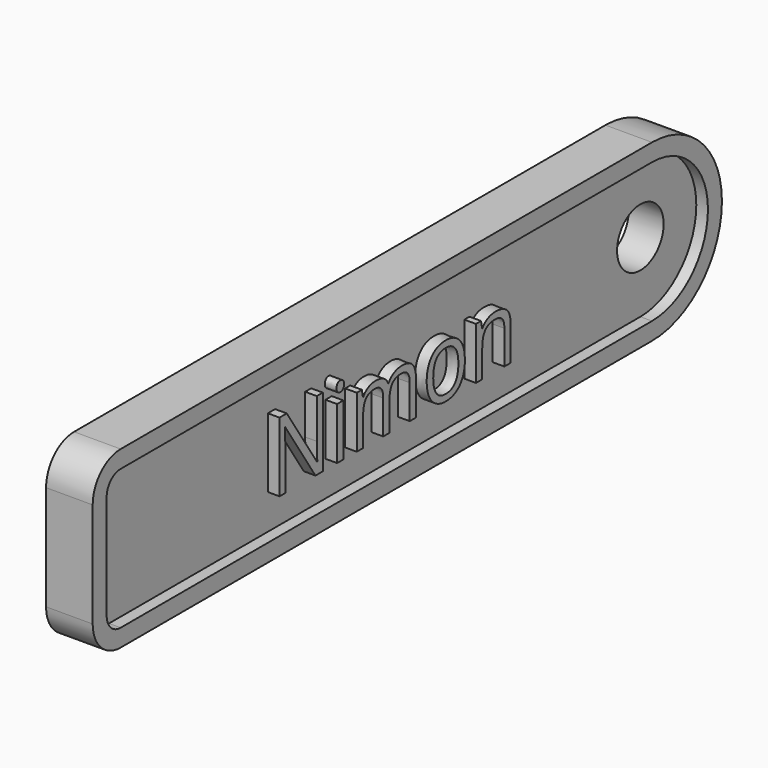
from build123d import *

# Parameters (mm, degrees)
F0_R         = 63.5
F1_DEPTH     = 76.2
F2_TEXT_SIZE = 211.6666666667
F3_DEPTH     = 25.4
F5_DEPTH     = 25.4


# Not quite as in the source:
# - Text() gives the source's letters only with a copy of the font that has no kerning and outlines rounded to 1/6400 em; it was checked with that copy


with BuildPart() as f1:
    # F0 (on Right) → F1 (new body)
    with BuildSketch(Plane.YZ):
        with BuildLine():
            Line((765.8453470916, 190.5), (-681.9546529084, 190.5))
            ThreePointArc((-681.9546529084, 190.5), (-735.8361896349, 168.1815367264), (-758.1546529084, 114.3))
            Line((-758.1546529084, 114.3), (-758.1546529084, -114.3))
            ThreePointArc((-758.1546529084, -114.3), (-735.8361896349, -168.1815367264), (-681.9546529084, -190.5))
            Line((-681.9546529084, -190.5), (765.8453470916, -190.5))
            ThreePointArc((765.8453470916, -190.5), (956.3453470916, 0), (765.8453470916, 190.5))
        make_face()
        with Locations((765.8453470916, 0)):
            Circle(F0_R, mode=Mode.SUBTRACT)
    extrude(amount=F1_DEPTH)

    # F2 (on face) → F3 (join)
    with BuildSketch(Plane.YZ.offset(76.2)):
        with Locations((-269.9523142815, -76.2)):
            Text('Nimon', F2_TEXT_SIZE, font='Open Sans', text_align=(TextAlign.LEFT, TextAlign.BOTTOM))
    extrude(amount=F3_DEPTH)

    # F4 (on face) → F5 (join)
    with BuildSketch(Plane.YZ.offset(76.2)):
        with BuildLine():
            ThreePointArc((-758.1546529084, -114.3), (-735.8361896349, -168.1815367264), (-681.9546529084, -190.5))
            Line((-681.9546529084, -190.5), (765.8453470916, -190.5))
            ThreePointArc((765.8453470916, -190.5), (956.3453470916, 0), (765.8453470916, 190.5))
            Line((765.8453470916, 190.5), (-681.9546529084, 190.5))
            ThreePointArc((-681.9546529084, 190.5), (-735.8361896349, 168.1815367264), (-758.1546529084, 114.3))
            Line((-758.1546529084, 114.3), (-758.1546529084, -114.3))
        make_face()
        with BuildLine():
            ThreePointArc((-720.0546529084, 114.3), (-708.8954212717, 141.2407683632), (-681.9546529084, 152.4))
            Line((-681.9546529084, 152.4), (765.8453470916, 152.4))
            ThreePointArc((765.8453470916, 152.4), (918.2453470916, 0), (765.8453470916, -152.4))
            Line((765.8453470916, -152.4), (-681.9546529084, -152.4))
            ThreePointArc((-681.9546529084, -152.4), (-708.8954212717, -141.2407683632), (-720.0546529084, -114.3))
            Line((-720.0546529084, -114.3), (-720.0546529084, 114.3))
        make_face(mode=Mode.SUBTRACT)
    extrude(amount=F5_DEPTH)


solid = f1.part
